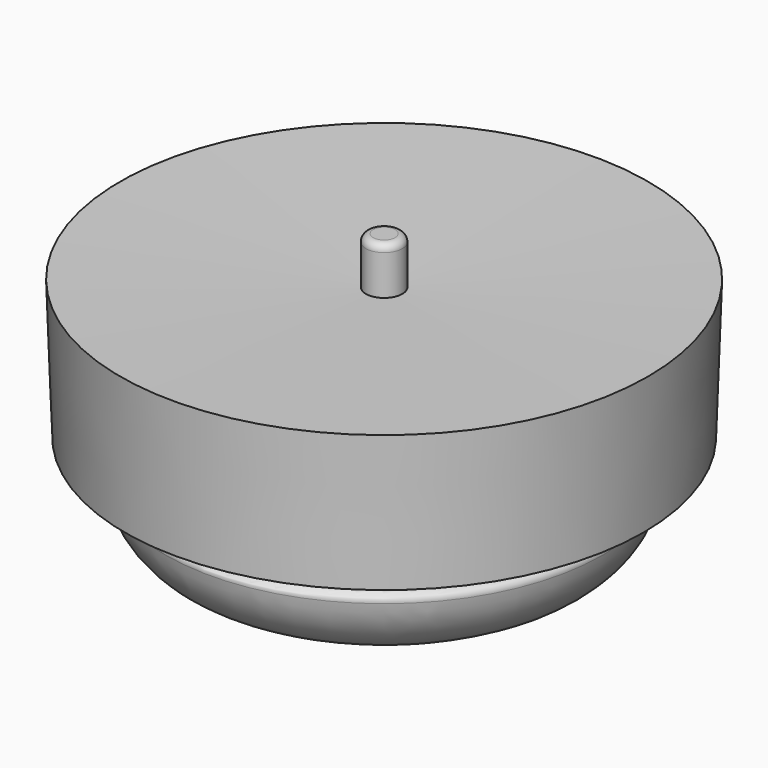
from build123d import *

# Parameters (mm, degrees)
F3_START = 12.7
F3_DEPTH = 19.05
F4_COUNT = 10


# Not quite as in the source:
# - a feature of the source that left no trace in its solid (it failed there, or was rolled back) is left out


with BuildPart() as f1:
    # F0 (on Front) → F1 (revolve)
    with BuildSketch(Plane.XZ):
        with BuildLine():
            Line((1.905, 50.8), (0, 50.8))
            Line((0, 50.8), (0, 3.429))
            ThreePointArc((0, 3.429), (1.234581103, 3.1990389963), (2.3035713577, 2.54))
            Line((2.3035713577, 2.54), (2.3283333333, 2.54))
            Line((2.3283333333, 2.54), (8.5069709166, 9.280331909))
            ThreePointArc((8.5069709166, 9.280331909), (11.6934487856, 10.4970314384), (14.5770403556, 8.6752469803))
            ThreePointArc((14.5770403556, 8.6752469803), (28.1700209381, 2.8349739515), (38.0701090446, 13.8288888889))
            ThreePointArc((38.0701090446, 13.8288888889), (37.7545750078, 14.8166666667), (36.8079728973, 15.24))
            Line((36.8079728973, 15.24), (11.2077643439, 15.24))
            ThreePointArc((11.2077643439, 15.24), (5.5147831679, 17.7339497654), (3.175, 23.492008017))
            Line((3.175, 23.492008017), (3.175, 28.447138482))
            Line((3.175, 28.447138482), (3.175, 42.5763448676))
            Line((3.175, 42.5763448676), (3.175, 49.53))
            ThreePointArc((3.175, 49.53), (2.8030256121, 50.4280256121), (1.905, 50.8))
        make_face()
    revolve(axis=Axis((0, 0, 27.1145), (0, 0, -1)))


with BuildPart() as f1b:
    # F0 (on Front) → F1, piece 2 (revolve)
    with BuildSketch(Plane.XZ):
        with BuildLine():
            Line((14.4074304519, 21.5152941176), (37.1261472623, 20.1133140583))
            ThreePointArc((37.1261472623, 20.1133140583), (37.0884679309, 20.290803038), (37.0258801512, 20.4611111111))
            ThreePointArc((37.0258801512, 20.4611111111), (26.8911688738, 27.8578215547), (15.3486127483, 22.9391737577))
            Line((15.3486127483, 22.9391737577), (14.4074304519, 21.5152941176))
        make_face()
    revolve(axis=Axis((0, 0, 27.1145), (0, 0, -1)))


with BuildPart() as f3:
    # F2 (on Top) → F3 (new body)
    with BuildSketch(Plane.XY.offset(F3_START)):
        with BuildLine():
            ThreePointArc((8.8605920386, 32.9803439023), (9.5332179712, 34.1474286699), (8.3661332036, 34.8200546025))
            ThreePointArc((8.3661332036, 34.8200546025), (-6.9590718106, 19.2711369672), (-0.8836379028, -1.6983611476))
            ThreePointArc((-0.8836379028, -1.6983611476), (0.4629208788, -1.6624174751), (0.4269772063, -0.3158586934))
            ThreePointArc((0.4269772063, -0.3158586934), (-5.1123890038, 18.8033895878), (8.8605920386, 32.9803439023))
        make_face()
    extrude(amount=F3_DEPTH)


with BuildPart() as f4_1:
    # F4: instance of F3
    add(f3.part.rotate(Axis((0, 0, 27.1145), (0, 0, -1)), 1 * 360 / F4_COUNT))


with BuildPart() as f4_2:
    # F4: instance of F3
    add(f3.part.rotate(Axis((0, 0, 27.1145), (0, 0, -1)), 2 * 360 / F4_COUNT))


with BuildPart() as f4_3:
    # F4: instance of F3
    add(f3.part.rotate(Axis((0, 0, 27.1145), (0, 0, -1)), 3 * 360 / F4_COUNT))


with BuildPart() as f4_4:
    # F4: instance of F3
    add(f3.part.rotate(Axis((0, 0, 27.1145), (0, 0, -1)), 4 * 360 / F4_COUNT))


with BuildPart() as f4_5:
    # F4: instance of F3
    add(f3.part.rotate(Axis((0, 0, 27.1145), (0, 0, -1)), 5 * 360 / F4_COUNT))


with BuildPart() as f4_6:
    # F4: instance of F3
    add(f3.part.rotate(Axis((0, 0, 27.1145), (0, 0, -1)), 6 * 360 / F4_COUNT))


with BuildPart() as f4_7:
    # F4: instance of F3
    add(f3.part.rotate(Axis((0, 0, 27.1145), (0, 0, -1)), 7 * 360 / F4_COUNT))


with BuildPart() as f4_8:
    # F4: instance of F3
    add(f3.part.rotate(Axis((0, 0, 27.1145), (0, 0, -1)), 8 * 360 / F4_COUNT))


with BuildPart() as f4_9:
    # F4: instance of F3
    add(f3.part.rotate(Axis((0, 0, 27.1145), (0, 0, -1)), 9 * 360 / F4_COUNT))


with BuildPart() as f5:
    # F0 (on Front) → F5 (revolve)
    with BuildSketch(Plane.XZ):
        with BuildLine():
            Line((14.4074304519, 21.5152941176), (37.1261472623, 20.1133140583))
            ThreePointArc((37.1261472623, 20.1133140583), (37.0884679309, 20.290803038), (37.0258801512, 20.4611111111))
            ThreePointArc((37.0258801512, 20.4611111111), (26.8911688738, 27.8578215547), (15.3486127483, 22.9391737577))
            Line((15.3486127483, 22.9391737577), (14.4074304519, 21.5152941176))
        make_face()
        with BuildLine():
            Line((46.0110940039, 43.8300818205), (3.175, 42.5763448676))
            Line((3.175, 42.5763448676), (3.175, 28.447138482))
            ThreePointArc((3.175, 28.447138482), (3.5303357558, 27.5660656584), (4.3975028668, 27.178026973))
            ThreePointArc((4.3975028668, 27.178026973), (9.3348579534, 25.9592138939), (13.3795915371, 22.8765022938))
            ThreePointArc((13.3795915371, 22.8765022938), (14.3790013058, 22.4397339438), (15.3486127483, 22.9391737577))
            ThreePointArc((15.3486127483, 22.9391737577), (26.8911688738, 27.8578215547), (37.0258801512, 20.4611111111))
            ThreePointArc((37.0258801512, 20.4611111111), (37.0884679309, 20.290803038), (37.1261472623, 20.1133140583))
            Line((37.1261472623, 20.1133140583), (45.1863929629, 19.6159134418))
            Line((45.1863929629, 19.6159134418), (46.0110940039, 43.8300818205))
        make_face()
    revolve(axis=Axis((0, 0, 27.1145), (0, 0, -1)))


solid = Compound([f1.part, f1b.part, f3.part, f4_1.part, f4_2.part, f4_3.part, f4_4.part, f4_5.part, f4_6.part, f4_7.part, f4_8.part, f4_9.part, f5.part])
